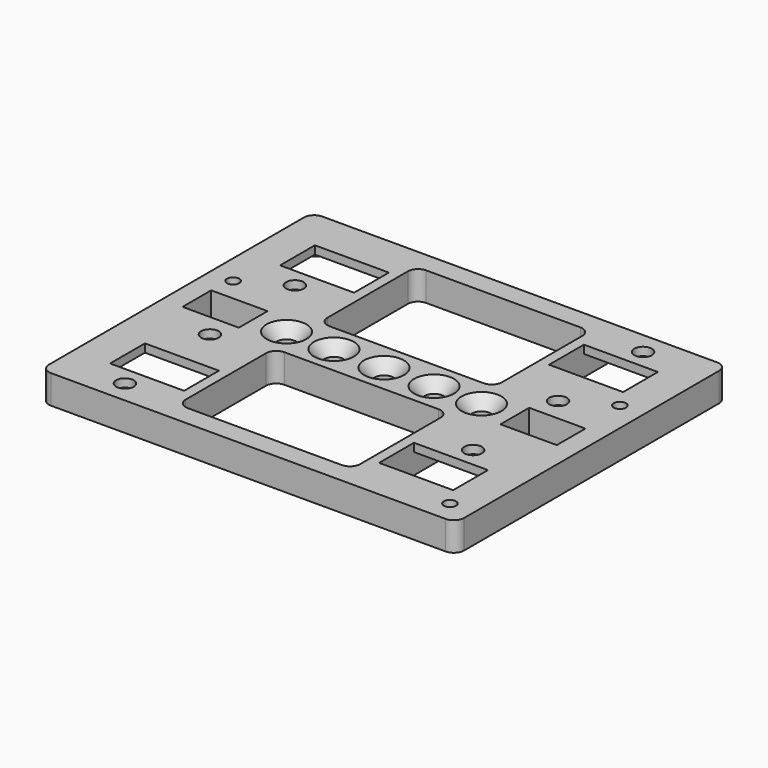
from build123d import *

# Parameters (mm, degrees)
F0_W           = 81.1
F0_H           = 66.25
F1_DEPTH       = 5.6
F3_D           = 3.45
F4_D           = 2.39
F6_D           = 3.7973
F6_CSINK_D     = 7.7978
F6_CSINK_ANGLE = 82
F8_DEPTH       = 3.9998
F7_W           = 34.1
F7_H           = 8.5
F7_W_2         = 14.45
F7_H_2         = 11
F7_W_3         = 11
F7_H_3         = 7
F7_H_4         = 4.125
F9_DEPTH       = 5.6
F10_R          = 2


with BuildPart() as f1:
    # F0 (on Top) → F1 (new body)
    with BuildSketch(Plane.XY):
        Rectangle(F0_W, F0_H)
    extrude(amount=F1_DEPTH)

    # F3 (through all)
    with Locations(Plane.XY.offset(5.6)):
        with Locations((-27.6, 12.75), (27.6, 28.75), (-27.6, -8), (27.6, 8), (27.6, -12.75), (-27.6, -28.75)):
            Hole(F3_D / 2)

    # F4 (through all)
    with Locations(Plane.XY.offset(5.6)):
        with Locations((-35.88, 8), (35.88, 12.75), (35.88, -28.75)):
            Hole(F4_D / 2)

    # F6 (through all)
    with Locations(Plane.XY.offset(5.6)):
        with Locations((0, 0), (-9.779, 0), (9.779, 0), (19.05, 0), (-19.05, 0)):
            CounterSinkHole(F6_D / 2, F6_CSINK_D / 2, counter_sink_angle=F6_CSINK_ANGLE)

    # F7 (on face) → F8 (cut, through all)
    with BuildSketch(Plane.XY):
        Polygon((-38.55, -5.5), (-38.55, -31.125), (-19.05, -31.125), (-19.05, -25), (-33.5, -25), (-33.5, -16.5), (-19.05, -16.5), (-19.05, -5.5), align=None)
        Polygon((-38.55, 31.125), (-38.55, 5.5), (-19.05, 5.5), (-19.05, 16.5), (-33.5, 16.5), (-33.5, 25), (-19.05, 25), (-19.05, 31.125), align=None)
        Polygon((19.05, 16.5), (19.05, 5.5), (38.55, 5.5), (38.55, 31.125), (19.05, 31.125), (19.05, 25), (33.5, 25), (33.5, 16.5), align=None)
        Polygon((19.05, -25), (19.05, -31.125), (38.55, -31.125), (38.55, -5.5), (19.05, -5.5), (19.05, -16.5), (33.5, -16.5), (33.5, -25), align=None)
    extrude(amount=F8_DEPTH, mode=Mode.SUBTRACT)

    # F7 (on face) → F9 (cut, through all)
    with BuildSketch(Plane.XY):
        with Locations((0, -20.75)):
            Rectangle(F7_W, F7_H)
        with Locations((0, 20.75)):
            Rectangle(F7_W, F7_H)
        with Locations((-26.275, -20.75)):
            Rectangle(F7_W_2, F7_H)
        with Locations((26.275, -20.75)):
            Rectangle(F7_W_2, F7_H)
        with Locations((26.275, 20.75)):
            Rectangle(F7_W_2, F7_H)
        with Locations((-26.275, 20.75)):
            Rectangle(F7_W_2, F7_H)
        with Locations((0, 11)):
            Rectangle(F7_W, F7_H_2)
        with Locations((0, -11)):
            Rectangle(F7_W, F7_H_2)
        with Locations((-31.05, 0)):
            Rectangle(F7_W_3, F7_H_3)
        with Locations((31.05, 0)):
            Rectangle(F7_W_3, F7_H_3)
        with Locations((0, 27.0625)):
            Rectangle(F7_W, F7_H_4)
        with Locations((0, -27.0625)):
            Rectangle(F7_W, F7_H_4)
    extrude(amount=F9_DEPTH, mode=Mode.SUBTRACT)

    # F10
    f10_edges = [f1.edges().sort_by_distance(p)[0] for p in [
        (-40.55, 33.125, 2.8),
        (40.55, 33.125, 2.8),
        (40.55, -33.125, 2.8),
        (-40.55, -33.125, 2.8),
        (-17.05, 5.5, 2.8),
        (17.05, 5.5, 2.8),
        (-17.05, -5.5, 2.8),
        (17.05, -5.5, 2.8),
        (38.55, 31.125, 1.9999),
        (38.55, -31.125, 1.9999),
        (-38.55, 31.125, 1.9999),
        (-38.55, -31.125, 1.9999),
        (-17.05, 29.125, 2.8),
        (17.05, 29.125, 2.8),
        (17.05, -29.125, 2.8),
        (-17.05, -29.125, 2.8),
    ]]
    fillet(f10_edges, radius=F10_R)


solid = f1.part
